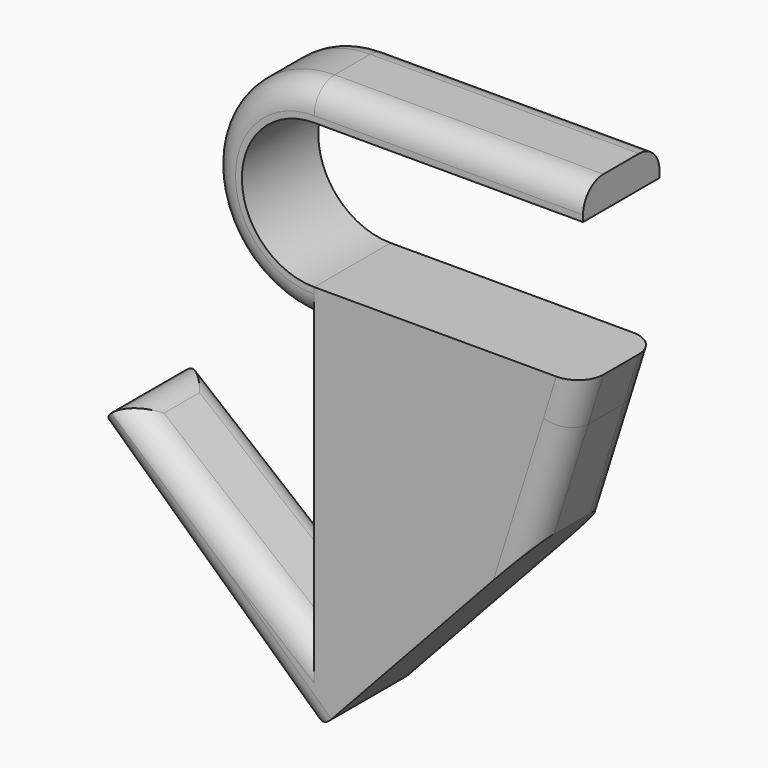
from build123d import *

# Parameters (mm, degrees)
F1_DEPTH    = 9.525
F2_R        = 5.08
F2_2_R      = 5.08
F3_T1_DEPTH = 44.45
F3_T3_DEPTH = 83.0687423867


# Not quite as in the source:
# - a fillet or chamfer that OpenCascade refuses, or shapes differently, is made with other operations: its cross-section is extruded or revolved along the edge and cut away or added


with BuildPart() as f1:
    # F0 (on Front) → F1 (new body, symmetric)
    with BuildSketch(Plane.XZ):
        Polygon((19.1333722323, 9.6779013216), (-34.4743542373, 9.6779013216), (-34.4743542373, 0), (16.0836418411, 0), align=None)
        Polygon((9.3244023705, -21.4495198637), (-34.4743542373, -21.4495198637), (-34.4743542373, -53.2785505056), (-34.4743542373, -68.7682205643), align=None)
        Polygon((-34.4743542373, -68.7682205643), (-34.4743542373, -53.2785505056), (-76.7960324883, -18.846389095), (-76.7960324883, -29.5947678383), align=None)
        Polygon((16.0836418411, 0), (-34.4743542373, 0), (-34.4743542373, -21.4495198637), (9.3244023705, -21.4495198637), align=None)
    extrude(amount=F1_DEPTH, both=True)

    # F2#2
    f2_2_edges = [f1.edges().sort_by_distance(p)[0] for p in [
        (-55.635193, -9.525, -36.06247),
        (-76.796032, 0, -18.846389),
        (-55.635193, 9.525, -36.06247),
        (14.228887, -9.525, -5.885809),
        (14.228887, 9.525, -5.885809),
    ]]
    fillet(f2_2_edges, radius=F2_2_R)

    # F3: fillet of radius 5.08 on 4 edges, made by hand

    # F3_s2 → F3_t1 (cut)
    with BuildSketch(Plane.XZ.offset(-22.225)):
        with BuildLine():
            ThreePointArc((-31.0235916298, -65.0401329276), (-34.5555808578, -66.6655840089), (-38.202441874, -65.3174579569))
            Line((-38.202441874, -65.3174579569), (-34.4743542373, -68.7682205643))
            Line((-34.4743542373, -68.7682205643), (-31.0235916298, -65.0401329276))
        make_face()
    extrude(amount=F3_T1_DEPTH, mode=Mode.SUBTRACT)

    # F3_s4 → F3_t3 (cut)
    with BuildSketch(Plane(origin=(-35.9272257857, 0, 33.2546708697), x_dir=(0, 1, 0), z_dir=(0.733875519, 0, -0.6792839778))):
        with BuildLine():
            ThreePointArc((-9.525, -68.8051900398), (-8.0371024484, -72.3972924882), (-4.445, -73.8851900398))
            Line((-4.445, -73.8851900398), (-9.525, -73.8851900398))
            Line((-9.525, -73.8851900398), (-9.525, -68.8051900398))
        make_face()
        with BuildLine():
            ThreePointArc((9.525, -68.8051900398), (8.0371024484, -72.3972924882), (4.445, -73.8851900398))
            Line((4.445, -73.8851900398), (9.525, -73.8851900398))
            Line((9.525, -73.8851900398), (9.525, -68.8051900398))
        make_face()
    extrude(amount=F3_T3_DEPTH, mode=Mode.SUBTRACT)


with BuildPart() as f1b:
    # F0 (on Front) → F1, piece 2 (new body, symmetric)
    with BuildSketch(Plane.XZ):
        with BuildLine():
            Line((-34.4743542373, 38.5207416654), (19.1333722323, 38.5207416654))
            Line((19.1333722323, 38.5207416654), (19.1333722323, 44.8707416654))
            Line((19.1333722323, 44.8707416654), (-34.4743542373, 44.8707416654))
            ThreePointArc((-34.4743542373, 44.8707416654), (-55.2457359555, 24.1392899111), (-34.5542909246, 3.3280551363))
            Line((-34.5542909246, 3.3280551363), (-34.4743542373, 9.6779013216))
            ThreePointArc((-34.4743542373, 9.6779013216), (-48.8957744092, 24.0993214935), (-34.4743542373, 38.5207416654))
        make_face()
    extrude(amount=F1_DEPTH, both=True)

    # F2
    f2_edges = [f1b.edges().sort_by_distance(p)[0] for p in [
        (-7.670491, -9.525, 44.870742),
        (-7.670491, 9.525, 44.870742),
    ]]
    fillet(f2_edges, radius=F2_R)


solid = Compound([f1.part, f1b.part])
